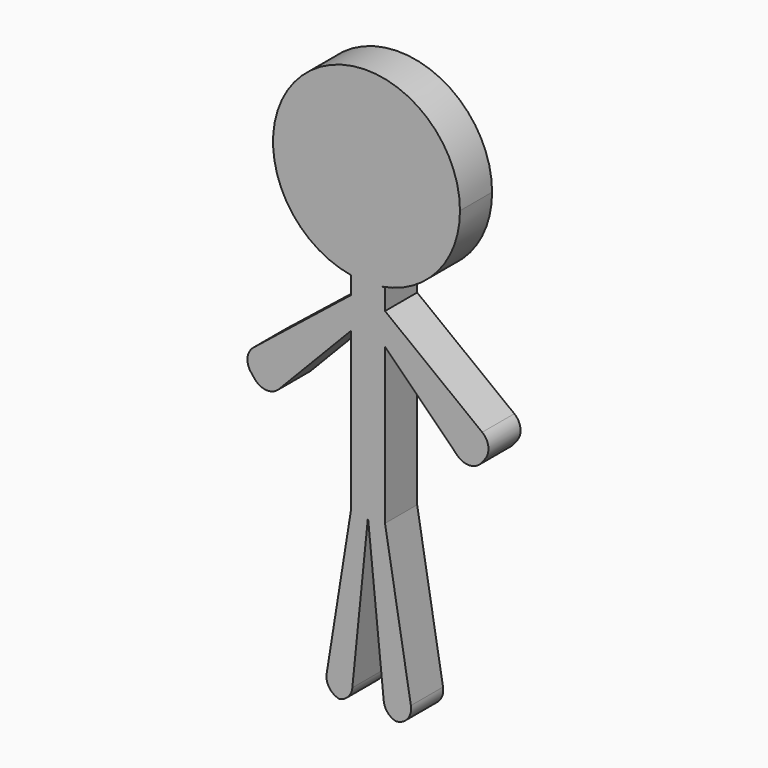
from build123d import *

# Parameters (mm, degrees)
F1_DEPTH     = 12.7
F2_T1_DEPTH  = 38.1
F2_T3_DEPTH  = 41.6542533238
F2_T5_DEPTH  = 41.5408544992
F2_T7_DEPTH  = 35.6725625774
F2_T9_DEPTH  = 33.4559034625
F2_T11_DEPTH = 42.4902813585
F2_T13_DEPTH = 46.0406969882


# Not quite as in the source:
# - a fillet or chamfer that OpenCascade refuses, or shapes differently, is made with other operations: its cross-section is extruded or revolved along the edge and cut away or added


with BuildPart() as f1:
    # F0 (on Front) → F1 (new body)
    with BuildSketch(Plane.XZ):
        with BuildLine():
            ThreePointArc((4.9426316758, 33.3698169468), (22.5960240749, 43.4449478875), (29.579706142, 62.5336542726))
            ThreePointArc((29.579706142, 62.5336542726), (-19.0887063851, 85.1296783474), (-4.9426316758, 33.3698169468))
            Line((-4.9426316758, 33.3698169468), (4.9426316758, 33.3698169468))
        make_face()
        with BuildLine():
            Line((4.9426316758, 33.3698169468), (-4.9426316758, 33.3698169468))
            ThreePointArc((-4.9426316758, 33.3698169468), (0, 32.9539481306), (4.9426316758, 33.3698169468))
        make_face()
        with BuildLine():
            ThreePointArc((4.9426316758, 33.3698169468), (0, 32.9539481306), (-4.9426316758, 33.3698169468))
            Line((-4.9426316758, 33.3698169468), (-4.9426316758, 27.7676489204))
            Line((-4.9426316758, 27.7676489204), (-4.9426316758, 17.8345050663))
            Line((-4.9426316758, 17.8345050663), (-4.9426316758, -32.282717526))
            Line((-4.9426316758, -32.282717526), (0.4634799664, -32.282717526))
            Line((0.4634799664, -32.282717526), (5.8695916086, -32.282717526))
            Line((5.8695916086, -32.282717526), (5.8695916086, 16.9314928353))
            Line((5.8695916086, 16.9314928353), (5.8695916086, 26.8646366894))
            Line((5.8695916086, 26.8646366894), (5.8695916086, 33.3698169468))
            Line((5.8695916086, 33.3698169468), (4.9426316758, 33.3698169468))
        make_face()
        Polygon((-4.9426316758, 17.8345050663), (-4.9426316758, 27.7676489204), (-39.732567966, 0), (-31.750221352, -10.0010386527), align=None)
        Polygon((40.6355895102, 0), (5.8695916086, 26.8646366894), (5.8695916086, 16.9314928353), (32.8805417262, -10.0359434636), align=None)
        Polygon((0.4634799664, -32.282717526), (-4.9426316758, -32.282717526), (-13.5451909155, -86.0119983554), (-4.9426316758, -86.0119983554), align=None)
        Polygon((5.8695916086, -32.282717526), (0.4634799664, -32.282717526), (5.8695916086, -86.0119983554), (15.1662486102, -86.9474057324), align=None)
    extrude(amount=F1_DEPTH)

    # F2: fillet of radius 5.08 on 8 edges, made by hand

    # F2_s2 → F2_t1 (cut)
    with BuildSketch(Plane.XZ.offset(-12.7)):
        with BuildLine():
            ThreePointArc((37.5294360638, -4.0197276981), (38.5484672449, -0.2675797032), (36.6158618121, 3.1061534464))
            Line((36.6158618121, 3.1061534464), (40.6355895102, 0))
            Line((40.6355895102, 0), (37.5294360638, -4.0197276981))
        make_face()
        with BuildLine():
            ThreePointArc((-35.7621773131, 3.168974292), (-37.641496387, -0.2347294175), (-36.5635936739, -3.9703906529))
            Line((-36.5635936739, -3.9703906529), (-39.732567966, 0))
            Line((-39.732567966, 0), (-35.7621773131, 3.168974292))
        make_face()
    extrude(amount=F2_T1_DEPTH, mode=Mode.SUBTRACT)

    # F2_s4 → F2_t3 (cut)
    with BuildSketch(Plane.XZ.offset(-14.4771266619)):
        with BuildLine():
            ThreePointArc((-35.3626341248, -5.4750663394), (-31.6283156718, -7.3806038383), (-27.7332133062, -5.8299958835))
            Line((-27.7332133062, -5.8299958835), (-31.750221352, -10.0010386527))
            Line((-31.750221352, -10.0010386527), (-35.3626341248, -5.4750663394))
        make_face()
    extrude(amount=F2_T3_DEPTH, mode=Mode.SUBTRACT)

    # F2_s6 → F2_t5 (cut)
    with BuildSketch(Plane.XZ.offset(-14.4204272496)):
        with BuildLine():
            ThreePointArc((28.7985423047, -5.960520019), (32.7134460909, -7.4350713917), (36.4074755687, -5.4716764688))
            Line((36.4074755687, -5.4716764688), (32.8805417262, -10.0359434636))
            Line((32.8805417262, -10.0359434636), (28.7985423047, -5.960520019))
        make_face()
    extrude(amount=F2_T5_DEPTH, mode=Mode.SUBTRACT)

    # F2_s8 → F2_t7 (cut)
    with BuildSketch(Plane.XZ.offset(-11.4862812887)):
        with BuildLine():
            ThreePointArc((-9.5371441912, -86.0119983554), (-6.1295888664, -84.699619184), (-4.4826652871, -81.4405679254))
            Line((-4.4826652871, -81.4405679254), (-4.9426316758, -86.0119983554))
            Line((-4.9426316758, -86.0119983554), (-9.5371441912, -86.0119983554))
        make_face()
    extrude(amount=F2_T7_DEPTH, mode=Mode.SUBTRACT)

    # F2_s10 → F2_t9 (cut)
    with BuildSketch(Plane.XZ.offset(-10.3779517312)):
        with BuildLine():
            ThreePointArc((5.4540081087, -81.8816725212), (6.9163845644, -84.9652053996), (9.9999174428, -86.4275818554))
            Line((9.9999174428, -86.4275818554), (5.8695916086, -86.0119983554))
            Line((5.8695916086, -86.0119983554), (5.4540081087, -81.8816725212))
        make_face()
    extrude(amount=F2_T9_DEPTH, mode=Mode.SUBTRACT)

    # F2_s12 → F2_t11 (cut)
    with BuildSketch(Plane.XZ.offset(-14.8951406792)):
        with BuildLine():
            ThreePointArc((-12.6032474685, -80.1288718839), (-11.452770586, -84.2279441623), (-7.5871346438, -86.0119983554))
            Line((-7.5871346438, -86.0119983554), (-13.5451909155, -86.0119983554))
            Line((-13.5451909155, -86.0119983554), (-12.6032474685, -80.1288718839))
        make_face()
    extrude(amount=F2_T11_DEPTH, mode=Mode.SUBTRACT)

    # F2_s14 → F2_t13 (cut)
    with BuildSketch(Plane.XZ.offset(-16.6703484941)):
        with BuildLine():
            ThreePointArc((8.5316088631, -86.2798441603), (12.7526164419, -84.6929586624), (14.0482707219, -80.3736542564))
            Line((14.0482707219, -80.3736542564), (15.1662486102, -86.9474057324))
            Line((15.1662486102, -86.9474057324), (8.5316088631, -86.2798441603))
        make_face()
    extrude(amount=F2_T13_DEPTH, mode=Mode.SUBTRACT)


solid = f1.part
